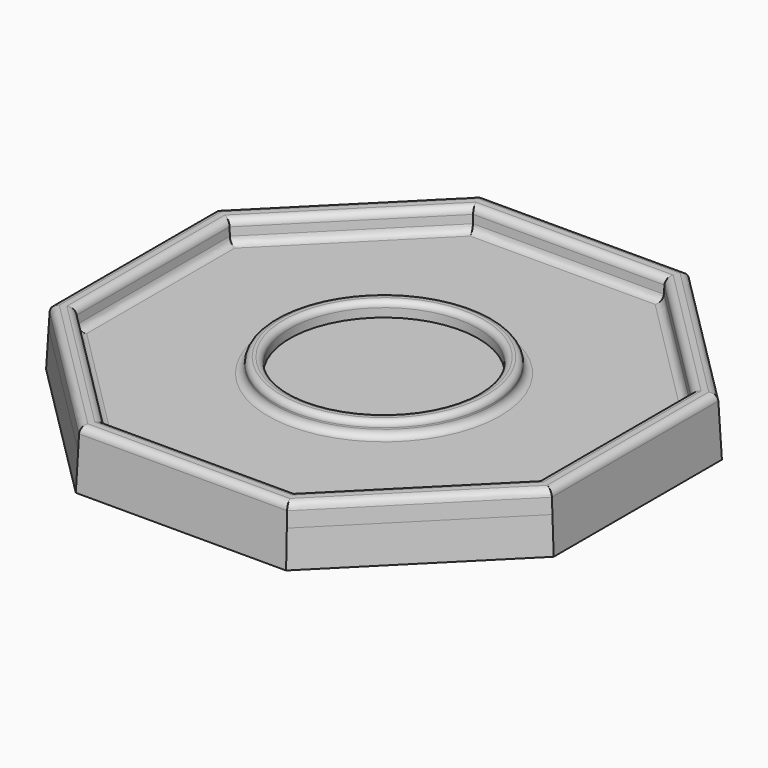
from build123d import *

# Parameters (mm, degrees)
F1_DEPTH = 5
F1_TAPER = 3
F3_DEPTH = 3
F3_TAPER = 3
F5_R     = 15
F5_R_2   = 13
F6_DEPTH = 2
F7_R     = 0.8
F8_R     = 1


# Not quite as in the source:
# - a feature of the source that left no trace in its solid (it failed there, or was rolled back) is left out


with BuildPart() as f1:
    # F0 (on Top) → F1 (new body)
    with BuildSketch(Plane.XY):
        Polygon((35, 14.4974746831), (14.4974746831, 35), (-14.4974746831, 35), (-35, 14.4974746831), (-35, -14.4974746831), (-14.4974746831, -35), (14.4974746831, -35), (35, -14.4974746831), align=None)
    extrude(amount=F1_DEPTH, taper=F1_TAPER)

    # F2 (on face) → F3 (join)
    with BuildSketch(Plane.XY.offset(5)):
        Polygon((34.7379611036, 14.3889346183), (14.3889346183, 34.7379611036), (-14.3889346183, 34.7379611036), (-34.7379611036, 14.3889346183), (-34.7379611036, -14.3889346183), (-14.3889346183, -34.7379611036), (14.3889346183, -34.7379611036), (34.7379611036, -14.3889346183), align=None)
        Polygon((13.1462939312, 31.7379611036), (31.7379611036, 13.1462939312), (31.7379611036, -13.1462939312), (13.1462939312, -31.7379611036), (-13.1462939312, -31.7379611036), (-31.7379611036, -13.1462939312), (-31.7379611036, 13.1462939312), (-13.1462939312, 31.7379611036), align=None, mode=Mode.SUBTRACT)
    extrude(amount=F3_DEPTH, taper=F3_TAPER)

    # F5 (on face) → F6 (join)
    with BuildSketch(Plane.XY.offset(5)):
        Circle(F5_R)
        Circle(F5_R_2, mode=Mode.SUBTRACT)
    extrude(amount=F6_DEPTH)

    # F7
    f7_edges = [f1.edges().sort_by_distance(p)[0] for p in [
        (-15, 0, 7),
        (-13, 0, 7),
    ]]
    fillet(f7_edges, radius=F7_R)

    # F8
    f8_edges = [f1.edges().sort_by_distance(p)[0] for p in [
        (-31.737961, 0, 5),
        (-22.442128, -22.442128, 5),
        (-22.442128, 22.442128, 5),
        (0, -31.737961, 5),
        (0, 31.737961, 5),
        (22.442128, -22.442128, 5),
        (22.442128, 22.442128, 5),
        (31.737961, 0, 5),
        (-15, 0, 5),
        (-31.895184, 0, 8),
        (-22.553301, -22.553301, 8),
        (-22.553301, 22.553301, 8),
        (0, -31.895184, 8),
        (0, 31.895184, 8),
        (22.553301, -22.553301, 8),
        (22.553301, 22.553301, 8),
        (31.895184, 0, 8),
        (34.580738, 0, 8),
        (24.452274, -24.452274, 8),
        (24.452274, 24.452274, 8),
        (0, -34.580738, 8),
        (0, 34.580738, 8),
        (-24.452274, -24.452274, 8),
        (-24.452274, 24.452274, 8),
        (-34.580738, 0, 8),
    ]]
    fillet(f8_edges, radius=F8_R)


solid = f1.part
